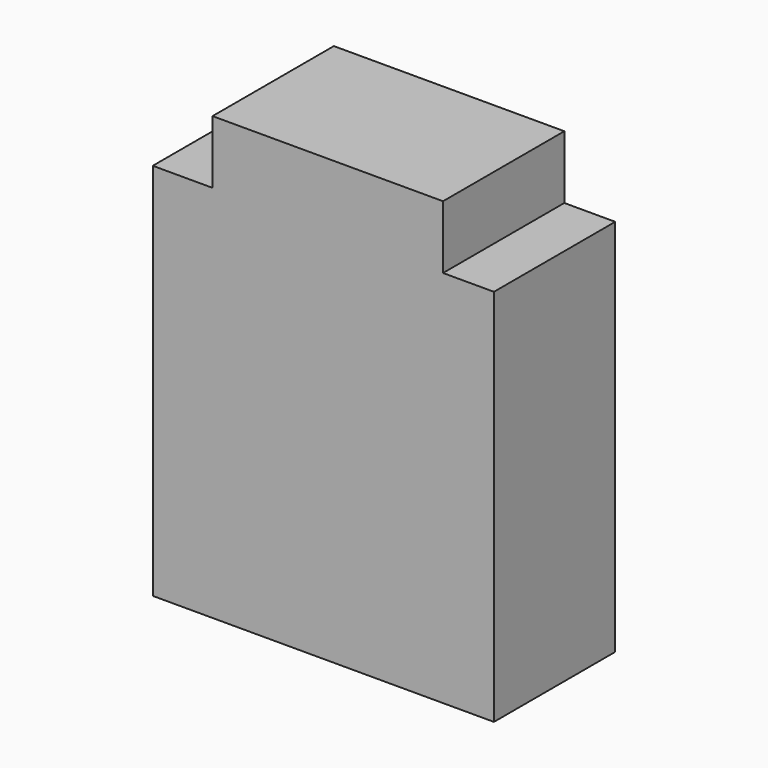
from build123d import *

# Parameters (mm, degrees)
F0_W       = 1371.6
F0_H       = 609.6
F1_DEPTH   = 254
F2_W       = 926.5377521515
F2_H       = 609.6
F1_FACE1_W = 1371.6
F1_FACE1_H = 609.6
F3_DEPTH   = 1522.3157249


# Not quite as in the source:
# - an extrude ends at something that could not be found from the text; its depth is read off the source's solid


with BuildPart() as f1:
    # F0 (on Top) → F1 (new body)
    with BuildSketch(Plane.XY):
        with Locations((54.0854626386, 40.4904214665)):
            Rectangle(F0_W, F0_H)
    extrude(amount=F1_DEPTH)

    # F2 (on face) + F1_face1 (on face) → F3 (join, through all)
    with BuildSketch(Plane.XY.offset(254)):
        with Locations((71.9089508057, 40.4904214665)):
            Rectangle(F2_W, F2_H)
    with BuildSketch(Plane(origin=(54.0854626386, 40.4904214665, 0), x_dir=(1, 0, 0), z_dir=(0, 0, -1))):
        Rectangle(F1_FACE1_W, F1_FACE1_H)
    extrude(amount=F3_DEPTH, dir=(0, 0, 1))


solid = f1.part
